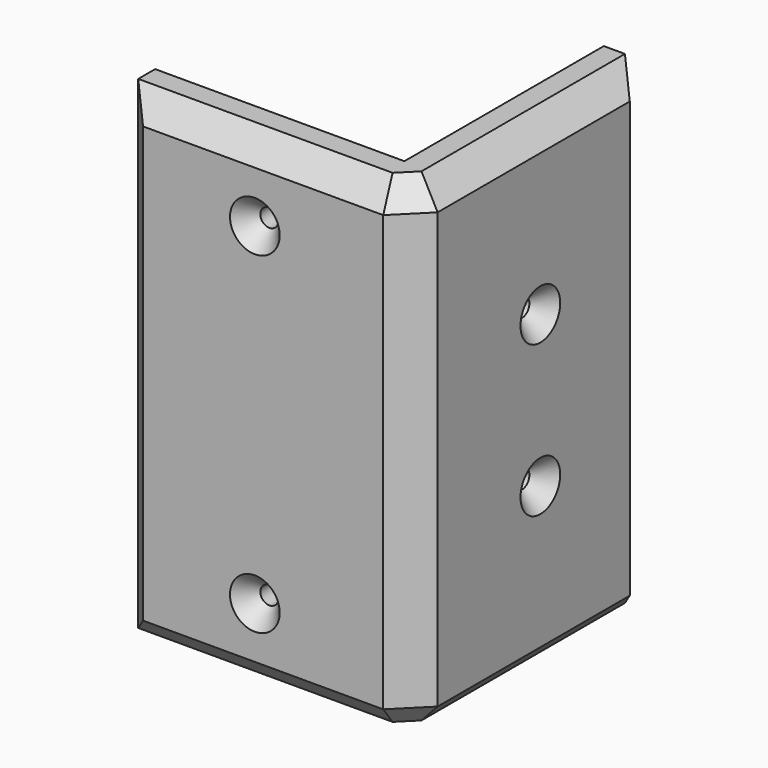
from build123d import *

# Parameters (mm, degrees)
F1_DEPTH             = 50.8
F3_DEPTH             = 50.8
F6_D                 = 3.7973
F6_CSINK_D           = 10.4394
F6_CSINK_ANGLE       = 82
F6_ON_F5_D           = 3.7973
F6_ON_F5_CSINK_D     = 10.4394
F6_ON_F5_CSINK_ANGLE = 82
F7_SIZE              = 6.35
F9_SIZE              = 5.08


# Not quite as in the source:
# - a feature of the source that left no trace in its solid (it failed there, or was rolled back) is left out
# - a feature names something its author has since deleted; it is built from what else it names


with BuildPart() as f1:
    # F0 (on Top) → F1 (new body)
    with BuildSketch(Plane.XY):
        Polygon((-61.9125, 0), (0, 0), (0, 61.9125), (-11.1125, 61.9125), (-11.1125, 11.1125), (-61.9125, 11.1125), align=None)
    extrude(amount=-F1_DEPTH)

    # F2 (on face) → F3 (join)
    with BuildSketch(Plane.XY):
        Polygon((0, 0), (0, 61.9125), (-9.525, 61.9125), (-9.525, 9.525), (-61.9125, 9.525), (-61.9125, 0), align=None)
    extrude(amount=F3_DEPTH)

    # F6 (through all)
    with Locations(Plane.YZ):
        with Locations((33.3375, -15.875), (33.3375, 15.875)):
            CounterSinkHole(F6_D / 2, F6_CSINK_D / 2, counter_sink_angle=F6_CSINK_ANGLE)

    # F6 on F5 (through all)
    with Locations(Plane.XZ):
        with Locations((-33.3375, 34.925), (-33.3375, -34.925)):
            CounterSinkHole(F6_ON_F5_D / 2, F6_ON_F5_CSINK_D / 2, counter_sink_angle=F6_ON_F5_CSINK_ANGLE)

    # F7
    f7_edges = [f1.edges().sort_by_distance(p)[0] for p in [
        (0, 0, 0),
    ]]
    chamfer(f7_edges, length=F7_SIZE)

    # F9
    f9_edges = [f1.edges().sort_by_distance(p)[0] for p in [
        (-34.13125, 0, 50.8),
        (-3.175, 3.175, 50.8),
        (0, 34.13125, 50.8),
        (-3.175, 3.175, -50.8),
        (-34.13125, 0, -50.8),
        (0, 34.13125, -50.8),
        (-61.9125, 0, 0),
        (0, 61.9125, 0),
    ]]
    chamfer(f9_edges, length=F9_SIZE)


solid = f1.part
